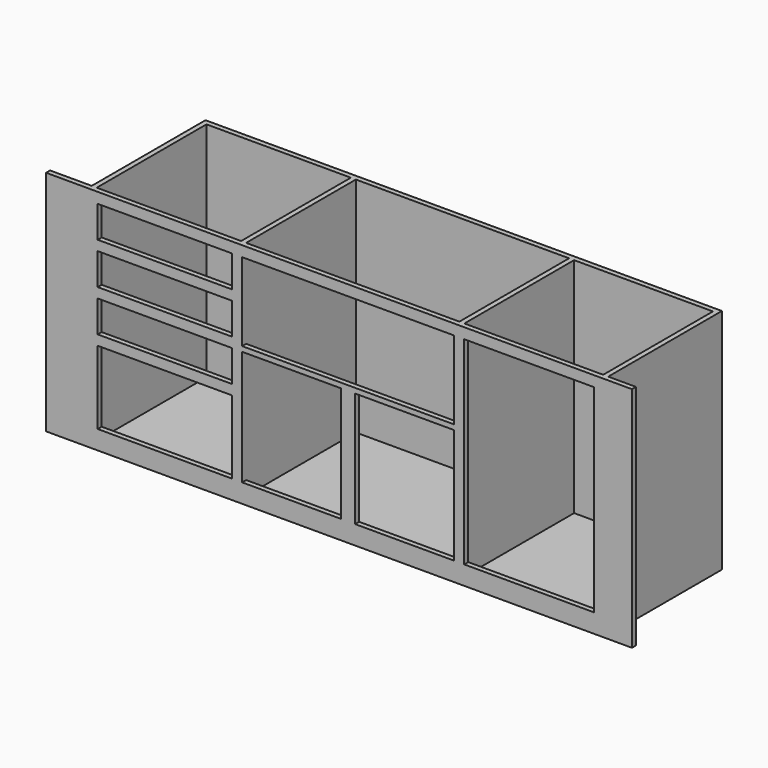
from build123d import *

# Parameters (mm, degrees)
F0_W     = 520
F0_H     = 494
F0_W_2   = 768
F0_W_3   = 500
F1_DEPTH = 820
F2_W     = 484
F2_H     = 114
F2_H_2   = 264
F2_W_2   = 357
F2_H_3   = 414
F3_DEPTH = 50
F4_W     = 1835.1259900331
F4_H     = 504.2004961409
F5_DEPTH = 18


# Not quite as in the source:
# - a feature names something its author has since deleted; it is built from what else it names


with BuildPart() as f1:
    # F0 (on Top) → F1 (new body)
    with BuildSketch(Plane.XY):
        Polygon((-150, 0), (0, 0), (1860, 0), (1960, 0), (1960, 18), (1860, 18), (1860, 530), (0, 530), (0, 18), (-150, 18), align=None)
        with Locations((278, 265)):
            Rectangle(F0_W, F0_H, mode=Mode.SUBTRACT)
        with Locations((940, 265)):
            Rectangle(F0_W_2, F0_H, mode=Mode.SUBTRACT)
        with Locations((1592, 265)):
            Rectangle(F0_W_3, F0_H, mode=Mode.SUBTRACT)
    extrude(amount=-F1_DEPTH)

    # F2 (on face) → F3 (cut)
    with BuildSketch(Plane.XZ):
        with Locations((278, -95)):
            Rectangle(F2_W, F2_H)
        with Locations((278, -245)):
            Rectangle(F2_W, F2_H)
        with Locations((278, -395)):
            Rectangle(F2_W, F2_H)
        with Locations((278, -620)):
            Rectangle(F2_W, F2_H_2)
        Polygon((556, -257.2889821529), (556, -320), (1320, -320), (1320, -38), (913, -38), (556, -38), align=None)
        with Locations((1141.5, -545)):
            Rectangle(F2_W_2, F2_H_3)
        Polygon((1572, -38), (1356, -38), (1356, -752), (1572, -752), (1608, -752), (1824, -752), (1824, -38), (1608, -38), align=None)
        Polygon((913, -338), (556, -338), (556, -407.2889821529), (556, -557.2889821529), (556, -752), (913, -752), align=None)
    extrude(amount=-F3_DEPTH, mode=Mode.SUBTRACT)

    # F4 (on face) → F5 (join)
    with BuildSketch(Plane(origin=(0, 0, -820), x_dir=(1, 0, 0), z_dir=(0, 0, -1))):
        with Locations((924.4370049834, -259.8997519296)):
            Rectangle(F4_W, F4_H)
    extrude(amount=-F5_DEPTH)


solid = f1.part
